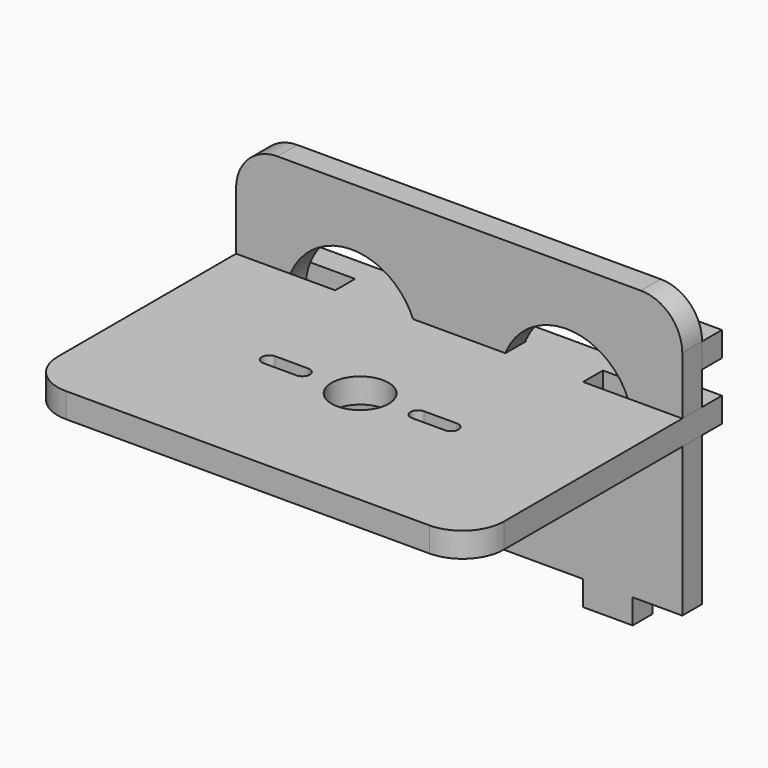
from build123d import *

# Parameters (mm, degrees)
F0_R     = 8
F1_DEPTH = 3
F2_W     = 54
F2_H     = 3
F3_DEPTH = 3
F4_R     = 3.45
F4_W     = 6
F4_H     = 3
F5_DEPTH = 3


# Not quite as in the source:
# - a feature names something its author has since deleted; it is built from what else it names


with BuildPart() as f1:
    # F0 (on Front) → F1 (new body)
    with BuildSketch(Plane.XZ):
        with BuildLine():
            Line((22, 15), (-22, 15))
            ThreePointArc((-22, 15), (-25.5355339059, 13.5355339059), (-27, 10))
            Line((-27, 10), (-27, -15))
            Line((-27, -15), (-27, -18))
            Line((-27, -18), (-21, -18))
            Line((-21, -18), (-21, -21))
            Line((-21, -21), (-15, -21))
            Line((-15, -21), (-15, -18))
            Line((-15, -18), (-9, -18))
            Line((-9, -18), (-3, -18))
            Line((-3, -18), (-1.5, -18))
            Line((-1.5, -18), (-1.5, -15))
            Line((-1.5, -15), (-3, -15))
            Line((-3, -15), (-3, -12.5))
            Line((-3, -12.5), (-1.5, -12.5))
            Line((-1.5, -12.5), (-1.5, -11))
            Line((-1.5, -11), (0, -11))
            Line((0, -11), (1.5, -11))
            Line((1.5, -11), (1.5, -12.5))
            Line((1.5, -12.5), (3, -12.5))
            Line((3, -12.5), (3, -15))
            Line((3, -15), (1.5, -15))
            Line((1.5, -15), (1.5, -18))
            Line((1.5, -18), (3, -18))
            Line((3, -18), (9, -18))
            Line((9, -18), (15, -18))
            Line((15, -18), (15, -21))
            Line((15, -21), (21, -21))
            Line((21, -21), (21, -18))
            Line((21, -18), (27, -18))
            Line((27, -18), (27, -15))
            Line((27, -15), (27, 10))
            ThreePointArc((27, 10), (25.5355339059, 13.5355339059), (22, 15))
        make_face()
        with Locations((-13, 0)):
            Circle(F0_R, mode=Mode.SUBTRACT)
        with Locations((13, 0)):
            Circle(F0_R, mode=Mode.SUBTRACT)
    extrude(amount=F1_DEPTH)


with BuildPart() as f3:
    # F2 (on face) → F3 (new body)
    with BuildSketch(Plane(origin=(0, 0, 0), x_dir=(-1, 0, 0), z_dir=(0, 1, 0))):
        with Locations((0, 8.5)):
            Rectangle(F2_W, F2_H)
    extrude(amount=F3_DEPTH)


with BuildPart() as f5:
    # F4 (on Top) → F5 (new body)
    with BuildSketch(Plane.XY):
        with BuildLine():
            Line((-27, 0), (-27, -3))
            Line((-27, -3), (-27, -30))
            ThreePointArc((-27, -30), (-25.5355339059, -33.5355339059), (-22, -35))
            Line((-22, -35), (22, -35))
            ThreePointArc((22, -35), (25.5355339059, -33.5355339059), (27, -30))
            Line((27, -30), (27, -3))
            Line((27, -3), (27, 0))
            Line((27, 0), (27, 3))
            Line((27, 3), (-27, 3))
            Line((-27, 3), (-27, 0))
        make_face()
        with BuildLine():
            Line((-7, -18.8810304218), (-11, -18.8810304218))
            ThreePointArc((-11, -18.8810304218), (-11.9, -17.9810304218), (-11, -17.0810304218))
            Line((-11, -17.0810304218), (-7, -17.0810304218))
            ThreePointArc((-7, -17.0810304218), (-6.1, -17.9810304218), (-7, -18.8810304218))
        make_face(mode=Mode.SUBTRACT)
        with Locations((0, -17.9810304218)):
            Circle(F4_R, mode=Mode.SUBTRACT)
        with BuildLine():
            ThreePointArc((11, -17.0810304218), (11.9, -17.9810304218), (11, -18.8810304218))
            Line((11, -18.8810304218), (7, -18.8798223013))
            ThreePointArc((7, -18.8798223013), (6.1012081205, -17.9810304218), (7, -17.0822385423))
            Line((7, -17.0822385423), (11, -17.0810304218))
        make_face(mode=Mode.SUBTRACT)
        with Locations((-18, -1.5)):
            Rectangle(F4_W, F4_H, mode=Mode.SUBTRACT)
        with BuildLine():
            ThreePointArc((0, 0), (1.0606601718, -0.4393398282), (1.5, -1.5))
            ThreePointArc((1.5, -1.5), (-1.0606601718, -2.5606601718), (0, 0))
        make_face(mode=Mode.SUBTRACT)
        with Locations((18, -1.5)):
            Rectangle(F4_W, F4_H, mode=Mode.SUBTRACT)
    extrude(amount=F5_DEPTH)


solid = Compound([f1.part, f3.part, f5.part])
